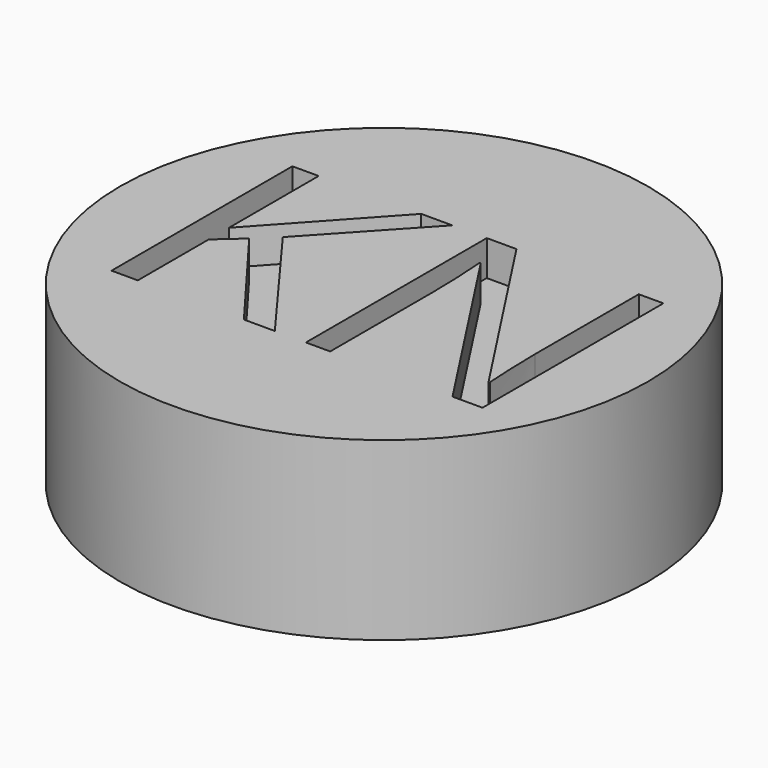
from build123d import *

# Parameters (mm, degrees)
F0_R         = 19.05
F2_DEPTH     = 12.7
F3_START     = 10.16
F1_TEXT_SIZE = 22.8421545667
F3_DEPTH     = 2.54


# Not quite as in the source:
# - Text() gives the source's letters only with a copy of the font that has no kerning and outlines rounded to 1/6400 em; it was checked with that copy


with BuildPart() as f2:
    # F0 (on Top) → F2 (new body)
    with BuildSketch(Plane.XY):
        Circle(F0_R)
    extrude(amount=F2_DEPTH)

    # F1 (on Top) → F3 (cut)
    with BuildSketch(Plane.XY.offset(F3_START)):
        with Locations((-15.24, -8.3183512881)):
            Text('KN', F1_TEXT_SIZE, font='Open Sans', text_align=(TextAlign.LEFT, TextAlign.BOTTOM))
    extrude(amount=F3_DEPTH, mode=Mode.SUBTRACT)


solid = f2.part
